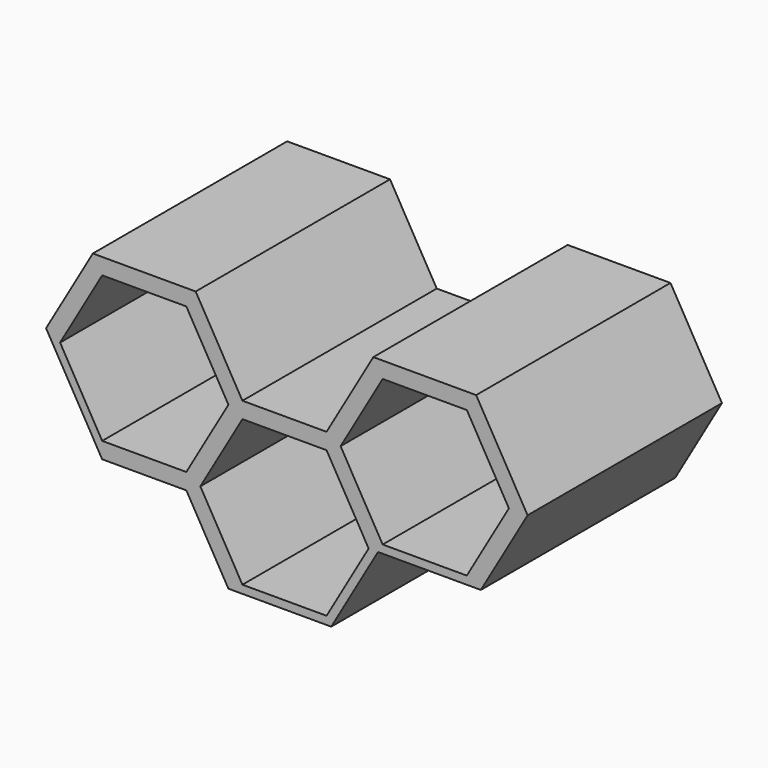
from build123d import *

# Parameters (mm, degrees)
F1_DEPTH = 12.7
F2_DEPTH = 95.25


# Not quite as in the source:
# - a feature names something its author has since deleted; it is built from what else it names


with BuildPart() as f1:
    # F0 (on Front) → F1 (new body)
    with BuildSketch(Plane.XZ):
        Polygon((-22.6091385288, 130.2924993012), (-4.278267482, 98.5424993012), (32.3834746115, 98.5424993012), (50.7143456583, 130.2924993012), (32.3834746116, 162.0424993012), (-4.278267482, 162.0424993012), align=None)
        Polygon((-2.4451803773, 101.7174993012), (-18.9429643194, 130.2924993012), (-2.4451803773, 158.8674993012), (30.5503875069, 158.8674993012), (47.048171449, 130.2924993012), (30.5503875069, 101.7174993012), align=None, mode=Mode.SUBTRACT)
        Polygon((-27.4963065598, 130.2924993012), (-22.6091385288, 130.2924993012), (-4.278267482, 162.0424993012), (-22.6091385288, 193.7924993012), (-59.2708806223, 193.7924993012), (-77.6017516691, 162.0424993012), (-59.2708806223, 130.2924993012), align=None)
        Polygon((-57.4377935176, 133.4674993012), (-73.9355774597, 162.0424993012), (-57.4377935176, 190.6174993012), (-24.4422256334, 190.6174993012), (-7.9444416913, 162.0424993012), (-24.4422256334, 133.4674993012), align=None, mode=Mode.SUBTRACT)
        Polygon((32.3834746116, 162.0424993012), (50.7143456583, 130.2924993012), (87.3760877519, 130.2924993012), (105.7069587986, 162.0424993012), (87.3760877519, 193.7924993012), (50.7143456583, 193.7924993012), align=None)
        Polygon((52.547432763, 133.4674993012), (36.0496488209, 162.0424993012), (52.547432763, 190.6174993012), (85.5430006472, 190.6174993012), (102.0407845893, 162.0424993012), (85.5430006472, 133.4674993012), align=None, mode=Mode.SUBTRACT)
        Polygon((-57.4377935176, 190.6174993012), (-73.9355774597, 162.0424993012), (-57.4377935176, 133.4674993012), (-24.4422256334, 133.4674993012), (-7.9444416913, 162.0424993012), (-24.4422256334, 190.6174993012), align=None)
        Polygon((52.547432763, 190.6174993012), (36.0496488209, 162.0424993012), (52.547432763, 133.4674993012), (85.5430006472, 133.4674993012), (102.0407845893, 162.0424993012), (85.5430006472, 190.6174993012), align=None)
        Polygon((-2.4451803773, 158.8674993012), (-18.9429643194, 130.2924993012), (-2.4451803773, 101.7174993012), (30.5503875069, 101.7174993012), (47.048171449, 130.2924993012), (30.5503875069, 158.8674993012), align=None)
    extrude(amount=F1_DEPTH)

    # F0 (on Front) → F2 (join)
    with BuildSketch(Plane.XZ):
        Polygon((-22.6091385288, 130.2924993012), (-4.278267482, 98.5424993012), (32.3834746115, 98.5424993012), (50.7143456583, 130.2924993012), (32.3834746116, 162.0424993012), (-4.278267482, 162.0424993012), align=None)
        Polygon((-2.4451803773, 101.7174993012), (-18.9429643194, 130.2924993012), (-2.4451803773, 158.8674993012), (30.5503875069, 158.8674993012), (47.048171449, 130.2924993012), (30.5503875069, 101.7174993012), align=None, mode=Mode.SUBTRACT)
        Polygon((32.3834746116, 162.0424993012), (50.7143456583, 130.2924993012), (87.3760877519, 130.2924993012), (105.7069587986, 162.0424993012), (87.3760877519, 193.7924993012), (50.7143456583, 193.7924993012), align=None)
        Polygon((52.547432763, 133.4674993012), (36.0496488209, 162.0424993012), (52.547432763, 190.6174993012), (85.5430006472, 190.6174993012), (102.0407845893, 162.0424993012), (85.5430006472, 133.4674993012), align=None, mode=Mode.SUBTRACT)
        Polygon((-27.4963065598, 130.2924993012), (-22.6091385288, 130.2924993012), (-4.278267482, 162.0424993012), (-22.6091385288, 193.7924993012), (-59.2708806223, 193.7924993012), (-77.6017516691, 162.0424993012), (-59.2708806223, 130.2924993012), align=None)
        Polygon((-57.4377935176, 133.4674993012), (-73.9355774597, 162.0424993012), (-57.4377935176, 190.6174993012), (-24.4422256334, 190.6174993012), (-7.9444416913, 162.0424993012), (-24.4422256334, 133.4674993012), align=None, mode=Mode.SUBTRACT)
        Polygon((-22.6091385288, 193.7924993012), (-4.278267482, 162.0424993012), (32.3834746116, 162.0424993012), (50.7143456583, 193.7924993012), (87.3760877519, 193.7924993012), (105.7069587986, 162.0424993012), (87.3760877519, 130.2924993012), (91.0422619612, 130.2924993012), (109.373133008, 162.0424993012), (89.2091748565, 196.9674993012), (48.8812585537, 196.9674993012), (30.5503875069, 165.2174993012), (-2.4451803773, 165.2174993012), (-20.7760514241, 196.9674993012), (-61.103967727, 196.9674993012), (-79.4348387737, 165.2174993012), (-77.6017516691, 162.0424993012), (-59.2708806223, 193.7924993012), align=None)
        Polygon((-7.9444416913, 98.5424993012), (-4.278267482, 98.5424993012), (-22.6091385288, 130.2924993012), (-27.4963065598, 130.2924993012), (-59.2708806223, 130.2924993012), (-57.4377935176, 127.1174993012), (-24.4422256334, 127.1174993012), align=None)
    extrude(amount=F2_DEPTH)


solid = f1.part
